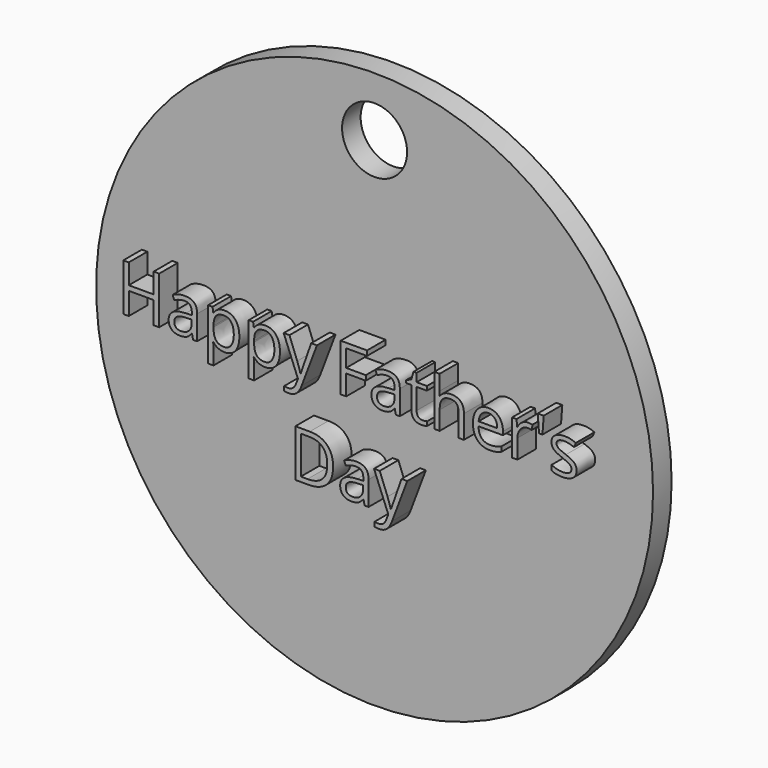
from build123d import *

# Parameters (mm, degrees)
F0_R         = 38.1
F1_DEPTH     = 3.175
F2_TEXT_SIZE = 9.0601034421
F3_DEPTH     = 3.175
F4_R         = 4.4487749904
F5_DEPTH     = 12.7


# Not quite as in the source:
# - Text() gives the source's letters only with a copy of the font that has no kerning and outlines rounded to 1/6400 em; it was checked with that copy


with BuildPart() as f1:
    # F0 (on Front) → F1 (new body)
    with BuildSketch(Plane.XZ):
        Circle(F0_R)
    extrude(amount=F1_DEPTH)

    # F2 (on face) → F3 (join)
    with BuildSketch(Plane.XZ.offset(3.175)):
        with Locations((-32.7321187408, 0)):
            Text("Happy Father's", F2_TEXT_SIZE, font='Open Sans', text_align=(TextAlign.LEFT, TextAlign.BOTTOM))
        with Locations((-9.1900062029, -12.3217406813)):
            Text('Day', F2_TEXT_SIZE, font='Open Sans', text_align=(TextAlign.LEFT, TextAlign.BOTTOM))
    extrude(amount=F3_DEPTH)

    # F4 (on face) → F5 (cut, symmetric)
    with BuildSketch(Plane.XZ.offset(3.175)):
        with Locations((0, 30.0185214728)):
            Circle(F4_R)
    extrude(amount=F5_DEPTH, both=True, mode=Mode.SUBTRACT)


solid = f1.part
